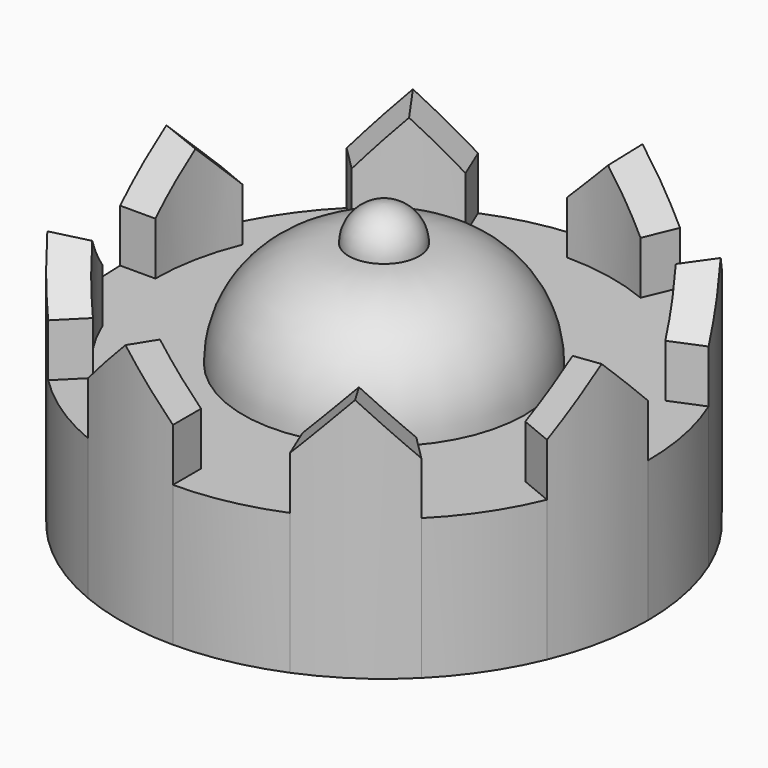
from build123d import *

# Parameters (mm, degrees)
F1_DEPTH     = 5.08
F2_DEPTH     = 8.89
F3_T1_DEPTH  = 11.0681121842
F3_T3_DEPTH  = 11.0681121842
F3_T5_DEPTH  = 11.0681121842
F3_T7_DEPTH  = 11.0681121842
F3_T9_DEPTH  = 11.0681121842
F3_T11_DEPTH = 11.0681121842
F3_T13_DEPTH = 11.0681121842
F3_T15_DEPTH = 11.0681121842
F3_T17_DEPTH = 11.0681121842
F3_T19_DEPTH = 11.0681121842
F3_T21_DEPTH = 11.0681121842
F3_T23_DEPTH = 11.0681121842
F3_T25_DEPTH = 11.0681121842
F3_T27_DEPTH = 11.0681121842
F3_T29_DEPTH = 11.0681121842
F3_T31_DEPTH = 11.0681121842
F4_R         = 5.08
F5_DEPTH     = 3.81
F6_R         = 3.80999
F7_R         = 1.27
F8_DEPTH     = 1.27
F9_R         = 1.26999


# Not quite as in the source:
# - a fillet or chamfer that OpenCascade refuses, or shapes differently, is made with other operations: its cross-section is extruded or revolved along the edge and cut away or added
# - a fillet or chamfer is up to 0.001 mm smaller than in the source, because OpenCascade refuses the exact size
# - a feature names something its author has since deleted; it is built from what else it names


with BuildPart() as f1:
    # F0 (on Top) → F1 (new body)
    with BuildSketch(Plane.XY):
        with BuildLine():
            Line((8.255, 0), (9.525, 0))
            ThreePointArc((9.525, 0), (9.3419797958, 1.8582353172), (8.7999525472, 3.6450596933))
            Line((8.7999525472, 3.6450596933), (7.6266255409, 3.1590517342))
            ThreePointArc((7.6266255409, 3.1590517342), (6.8637816496, 4.5862322736), (5.8371664787, 5.8371664787))
            Line((5.8371664787, 5.8371664787), (6.7351920908, 6.7351920908))
            ThreePointArc((6.7351920908, 6.7351920908), (5.2918064695, 7.9197480572), (3.6450596933, 8.7999525472))
            Line((3.6450596933, 8.7999525472), (3.1590517342, 7.6266255409))
            ThreePointArc((3.1590517342, 7.6266255409), (1.6104706082, 8.0963824897), (0, 8.255))
            Line((0, 8.255), (0, 9.525))
            ThreePointArc((0, 9.525), (-1.8582353172, 9.3419797958), (-3.6450596933, 8.7999525472))
            Line((-3.6450596933, 8.7999525472), (-3.1590517342, 7.6266255409))
            ThreePointArc((-3.1590517342, 7.6266255409), (-4.5862322736, 6.8637816496), (-5.8371664787, 5.8371664787))
            Line((-5.8371664787, 5.8371664787), (-6.7351920908, 6.7351920908))
            ThreePointArc((-6.7351920908, 6.7351920908), (-7.9197480572, 5.2918064695), (-8.7999525472, 3.6450596933))
            Line((-8.7999525472, 3.6450596933), (-7.6266255409, 3.1590517342))
            ThreePointArc((-7.6266255409, 3.1590517342), (-8.0963824897, 1.6104706082), (-8.255, 0))
            Line((-8.255, 0), (-9.525, 0))
            ThreePointArc((-9.525, 0), (-9.3419797958, -1.8582353172), (-8.7999525472, -3.6450596933))
            Line((-8.7999525472, -3.6450596933), (-7.6266255409, -3.1590517342))
            ThreePointArc((-7.6266255409, -3.1590517342), (-6.8637816496, -4.5862322736), (-5.8371664787, -5.8371664787))
            Line((-5.8371664787, -5.8371664787), (-6.7351920908, -6.7351920908))
            ThreePointArc((-6.7351920908, -6.7351920908), (-5.2918064695, -7.9197480572), (-3.6450596933, -8.7999525472))
            Line((-3.6450596933, -8.7999525472), (-3.1590517342, -7.6266255409))
            ThreePointArc((-3.1590517342, -7.6266255409), (-1.6104706082, -8.0963824897), (0, -8.255))
            Line((0, -8.255), (0, -9.525))
            ThreePointArc((0, -9.525), (1.8582353172, -9.3419797958), (3.6450596933, -8.7999525472))
            Line((3.6450596933, -8.7999525472), (3.1590517342, -7.6266255409))
            ThreePointArc((3.1590517342, -7.6266255409), (4.5862322736, -6.8637816496), (5.8371664787, -5.8371664787))
            Line((5.8371664787, -5.8371664787), (6.7351920908, -6.7351920908))
            ThreePointArc((6.7351920908, -6.7351920908), (7.9197480572, -5.2918064695), (8.7999525472, -3.6450596933))
            Line((8.7999525472, -3.6450596933), (7.6266255409, -3.1590517342))
            ThreePointArc((7.6266255409, -3.1590517342), (8.0963824897, -1.6104706082), (8.255, 0))
        make_face()
        with BuildLine():
            ThreePointArc((-8.7999525472, -3.6450596933), (-7.9197480572, -5.2918064695), (-6.7351920908, -6.7351920908))
            Line((-6.7351920908, -6.7351920908), (-5.8371664787, -5.8371664787))
            ThreePointArc((-5.8371664787, -5.8371664787), (-6.8637816496, -4.5862322736), (-7.6266255409, -3.1590517342))
            Line((-7.6266255409, -3.1590517342), (-8.7999525472, -3.6450596933))
        make_face()
    extrude(amount=F1_DEPTH)

    # F0 (on Top) → F2 (join)
    with BuildSketch(Plane.XY):
        with BuildLine():
            Line((3.1590517342, 7.6266255409), (3.6450596933, 8.7999525472))
            ThreePointArc((3.6450596933, 8.7999525472), (1.8582353172, 9.3419797958), (0, 9.525))
            Line((0, 9.525), (0, 8.255))
            ThreePointArc((0, 8.255), (1.6104706082, 8.0963824897), (3.1590517342, 7.6266255409))
        make_face()
        with BuildLine():
            Line((7.6266255409, 3.1590517342), (8.7999525472, 3.6450596933))
            ThreePointArc((8.7999525472, 3.6450596933), (7.9197480572, 5.2918064695), (6.7351920908, 6.7351920908))
            Line((6.7351920908, 6.7351920908), (5.8371664787, 5.8371664787))
            ThreePointArc((5.8371664787, 5.8371664787), (6.8637816496, 4.5862322736), (7.6266255409, 3.1590517342))
        make_face()
        with BuildLine():
            ThreePointArc((3.6450596933, -8.7999525472), (5.2918064695, -7.9197480572), (6.7351920908, -6.7351920908))
            Line((6.7351920908, -6.7351920908), (5.8371664787, -5.8371664787))
            ThreePointArc((5.8371664787, -5.8371664787), (4.5862322736, -6.8637816496), (3.1590517342, -7.6266255409))
            Line((3.1590517342, -7.6266255409), (3.6450596933, -8.7999525472))
        make_face()
        with BuildLine():
            ThreePointArc((8.7999525472, -3.6450596933), (9.3419797958, -1.8582353172), (9.525, 0))
            Line((9.525, 0), (8.255, 0))
            ThreePointArc((8.255, 0), (8.0963824897, -1.6104706082), (7.6266255409, -3.1590517342))
            Line((7.6266255409, -3.1590517342), (8.7999525472, -3.6450596933))
        make_face()
        with BuildLine():
            ThreePointArc((-3.6450596933, -8.7999525472), (-1.8582353172, -9.3419797958), (0, -9.525))
            Line((0, -9.525), (0, -8.255))
            ThreePointArc((0, -8.255), (-1.6104706082, -8.0963824897), (-3.1590517342, -7.6266255409))
            Line((-3.1590517342, -7.6266255409), (-3.6450596933, -8.7999525472))
        make_face()
        with BuildLine():
            ThreePointArc((-8.7999525472, -3.6450596933), (-7.9197480572, -5.2918064695), (-6.7351920908, -6.7351920908))
            Line((-6.7351920908, -6.7351920908), (-5.8371664787, -5.8371664787))
            ThreePointArc((-5.8371664787, -5.8371664787), (-6.8637816496, -4.5862322736), (-7.6266255409, -3.1590517342))
            Line((-7.6266255409, -3.1590517342), (-8.7999525472, -3.6450596933))
        make_face()
        with BuildLine():
            Line((-7.6266255409, 3.1590517342), (-8.7999525472, 3.6450596933))
            ThreePointArc((-8.7999525472, 3.6450596933), (-9.3419797958, 1.8582353172), (-9.525, 0))
            Line((-9.525, 0), (-8.255, 0))
            ThreePointArc((-8.255, 0), (-8.0963824897, 1.6104706082), (-7.6266255409, 3.1590517342))
        make_face()
        with BuildLine():
            Line((-3.1590517342, 7.6266255409), (-3.6450596933, 8.7999525472))
            ThreePointArc((-3.6450596933, 8.7999525472), (-5.2918064695, 7.9197480572), (-6.7351920908, 6.7351920908))
            Line((-6.7351920908, 6.7351920908), (-5.8371664787, 5.8371664787))
            ThreePointArc((-5.8371664787, 5.8371664787), (-4.5862322736, 6.8637816496), (-3.1590517342, 7.6266255409))
        make_face()
    extrude(amount=F2_DEPTH)

    # F3: chamfer of 1.905 on 16 edges, made by hand

    # F3_s2 → F3_t1 (cut)
    with BuildSketch(Plane(origin=(1.2842641335, 3.1004878888, 0), x_dir=(0, 0, 1), z_dir=(0.3826834324, 0.9238795325, 0))):
        Polygon((8.89, -1.905), (6.985, 0), (8.89, 0), align=None)
    extrude(amount=F3_T1_DEPTH, mode=Mode.SUBTRACT)

    # F3_s4 → F3_t3 (cut)
    with BuildSketch(Plane.XZ.offset(-14.4240560921)):
        Polygon((0, 6.985), (1.905, 8.89), (0, 8.89), align=None)
    extrude(amount=F3_T3_DEPTH, mode=Mode.SUBTRACT)

    # F3_s6 → F3_t5 (cut)
    with BuildSketch(Plane(origin=(3.1004878888, 1.2842641335, 0), x_dir=(0, 0, 1), z_dir=(0.9238795325, 0.3826834324, 0))):
        Polygon((8.89, -1.905), (6.985, 0), (8.89, 0), align=None)
    extrude(amount=F3_T5_DEPTH, mode=Mode.SUBTRACT)

    # F3_s8 → F3_t7 (cut)
    with BuildSketch(Plane(origin=(10.1993478749, 10.1993478749, 0), x_dir=(0, 0, 1), z_dir=(-0.7071067812, -0.7071067812, 0))):
        Polygon((6.985, 0), (8.89, -1.905), (8.89, 0), align=None)
    extrude(amount=F3_T7_DEPTH, mode=Mode.SUBTRACT)

    # F3_s10 → F3_t9 (cut)
    with BuildSketch(Plane(origin=(1.2842641335, -3.1004878888, 0), x_dir=(0, 0, 1), z_dir=(0.3826834324, -0.9238795325, 0))):
        Polygon((8.89, -1.905), (6.985, 0), (8.89, 0), align=None)
    extrude(amount=F3_T9_DEPTH, mode=Mode.SUBTRACT)

    # F3_s12 → F3_t11 (cut)
    with BuildSketch(Plane(origin=(10.1993478749, -10.1993478749, 0), x_dir=(0, 0, 1), z_dir=(-0.7071067812, 0.7071067812, 0))):
        Polygon((6.985, 0), (8.89, -1.905), (8.89, 0), align=None)
    extrude(amount=F3_T11_DEPTH, mode=Mode.SUBTRACT)

    # F3_s14 → F3_t13 (cut)
    with BuildSketch(Plane(origin=(3.1004878888, -1.2842641335, 0), x_dir=(0, 0, 1), z_dir=(0.9238795325, -0.3826834324, 0))):
        Polygon((8.89, -1.905), (6.985, 0), (8.89, 0), align=None)
    extrude(amount=F3_T13_DEPTH, mode=Mode.SUBTRACT)

    # F3_s16 → F3_t15 (cut)
    with BuildSketch(Plane.YZ.offset(3.3559439079)):
        Polygon((0, 6.985), (-1.905, 8.89), (0, 8.89), align=None)
    extrude(amount=F3_T15_DEPTH, mode=Mode.SUBTRACT)

    # F3_s18 → F3_t17 (cut)
    with BuildSketch(Plane.XZ.offset(3.3559439079)):
        Polygon((0, 6.985), (-1.905, 8.89), (0, 8.89), align=None)
    extrude(amount=F3_T17_DEPTH, mode=Mode.SUBTRACT)

    # F3_s20 → F3_t19 (cut)
    with BuildSketch(Plane(origin=(-1.2842641335, -3.1004878888, 0), x_dir=(0, 0, 1), z_dir=(-0.3826834324, -0.9238795325, 0))):
        Polygon((8.89, -1.905), (6.985, 0), (8.89, 0), align=None)
    extrude(amount=F3_T19_DEPTH, mode=Mode.SUBTRACT)

    # F3_s22 → F3_t21 (cut)
    with BuildSketch(Plane(origin=(-10.1993478749, -10.1993478749, 0), x_dir=(0, 0, 1), z_dir=(0.7071067812, 0.7071067812, 0))):
        Polygon((6.985, 0), (8.89, -1.905), (8.89, 0), align=None)
    extrude(amount=F3_T21_DEPTH, mode=Mode.SUBTRACT)

    # F3_s24 → F3_t23 (cut)
    with BuildSketch(Plane(origin=(-3.1004878888, -1.2842641335, 0), x_dir=(0, 0, 1), z_dir=(-0.9238795325, -0.3826834324, 0))):
        Polygon((8.89, -1.905), (6.985, 0), (8.89, 0), align=None)
    extrude(amount=F3_T23_DEPTH, mode=Mode.SUBTRACT)

    # F3_s26 → F3_t25 (cut)
    with BuildSketch(Plane.YZ.offset(-14.4240560921)):
        Polygon((0, 6.985), (1.905, 8.89), (0, 8.89), align=None)
    extrude(amount=F3_T25_DEPTH, mode=Mode.SUBTRACT)

    # F3_s28 → F3_t27 (cut)
    with BuildSketch(Plane(origin=(-3.1004878888, 1.2842641335, 0), x_dir=(0, 0, 1), z_dir=(-0.9238795325, 0.3826834324, 0))):
        Polygon((8.89, -1.905), (6.985, 0), (8.89, 0), align=None)
    extrude(amount=F3_T27_DEPTH, mode=Mode.SUBTRACT)

    # F3_s30 → F3_t29 (cut)
    with BuildSketch(Plane(origin=(-10.1993478749, 10.1993478749, 0), x_dir=(0, 0, 1), z_dir=(0.7071067812, -0.7071067812, 0))):
        Polygon((6.985, 0), (8.89, -1.905), (8.89, 0), align=None)
    extrude(amount=F3_T29_DEPTH, mode=Mode.SUBTRACT)

    # F3_s32 → F3_t31 (cut)
    with BuildSketch(Plane(origin=(-1.2842641335, 3.1004878888, 0), x_dir=(0, 0, 1), z_dir=(-0.3826834324, 0.9238795325, 0))):
        Polygon((8.89, -1.905), (6.985, 0), (8.89, 0), align=None)
    extrude(amount=F3_T31_DEPTH, mode=Mode.SUBTRACT)

    # F4 (on face) → F5 (join)
    with BuildSketch(Plane.XY.offset(5.08)):
        Circle(F4_R)
    extrude(amount=F5_DEPTH)

    # F6 (radius 3.81 in the source; OpenCascade refuses exactly that, so slightly less here)
    f6_edges = [f1.edges().sort_by_distance(p)[0] for p in [
        (-5.08, 0, 8.89),
    ]]
    fillet(f6_edges, radius=F6_R)

    # F7 (on face) → F8 (join)
    with BuildSketch(Plane.XY.offset(8.89)):
        Circle(F7_R)
    extrude(amount=F8_DEPTH)

    # F9 (radius 1.27 in the source; OpenCascade refuses exactly that, so slightly less here)
    f9_edges = [f1.edges().sort_by_distance(p)[0] for p in [
        (-1.27, 0, 10.16),
    ]]
    fillet(f9_edges, radius=F9_R)


solid = f1.part
